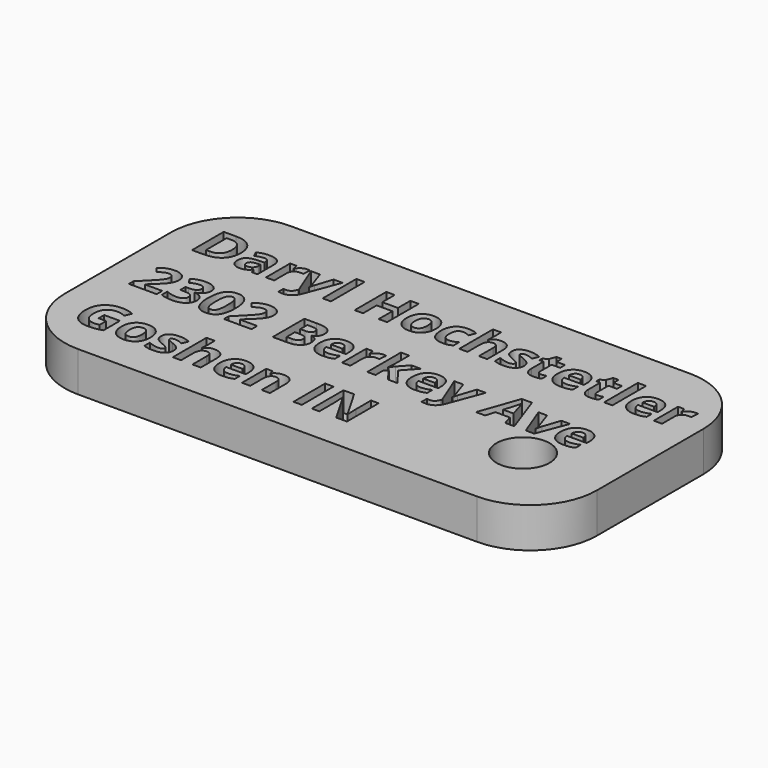
from build123d import *

# Parameters (mm, degrees)
F0_W         = 101.6
F0_H         = 50.8
F1_DEPTH     = 7.62
F2_TEXT_SIZE = 10.5833333333
F3_DEPTH     = 3.81
F4_R         = 5.08
F5_DEPTH     = 7.621
F6_R         = 12.7


# Not quite as in the source:
# - Text() gives the source's letters only with a copy of the font that has no kerning and outlines rounded to 1/6400 em; it was checked with that copy


with BuildPart() as f1:
    # F0 (on Top) → F1 (new body)
    with BuildSketch(Plane.XY):
        Rectangle(F0_W, F0_H)
    extrude(amount=F1_DEPTH)

    # F2 (on face) → F3 (cut)
    with BuildSketch(Plane.XY.offset(7.62)):
        with Locations((-45.72, 10.16)):
            Text('Daryl Hochstetler', F2_TEXT_SIZE, font='Open Sans', font_style=FontStyle.BOLD, text_align=(TextAlign.LEFT, TextAlign.BOTTOM))
        with Locations((-45.72, -4.2333333333)):
            Text('2302 Berkey Ave', F2_TEXT_SIZE, font='Open Sans', font_style=FontStyle.BOLD, text_align=(TextAlign.LEFT, TextAlign.BOTTOM))
        with Locations((-45.72, -18.6266666667)):
            Text('Goshen IN', F2_TEXT_SIZE, font='Open Sans', font_style=FontStyle.BOLD, text_align=(TextAlign.LEFT, TextAlign.BOTTOM))
    extrude(amount=-F3_DEPTH, mode=Mode.SUBTRACT)

    # F4 (on face) → F5 (cut, through all)
    with BuildSketch(Plane.XY.offset(7.62)):
        with Locations((34.6637239583, -10.16)):
            Circle(F4_R)
    extrude(amount=-F5_DEPTH, mode=Mode.SUBTRACT)

    # F6
    f6_edges = [f1.edges().sort_by_distance(p)[0] for p in [
        (-50.8, 25.4, 3.81),
        (-50.8, -25.4, 3.81),
        (50.8, 25.4, 3.81),
        (50.8, -25.4, 3.81),
    ]]
    fillet(f6_edges, radius=F6_R)


solid = f1.part
